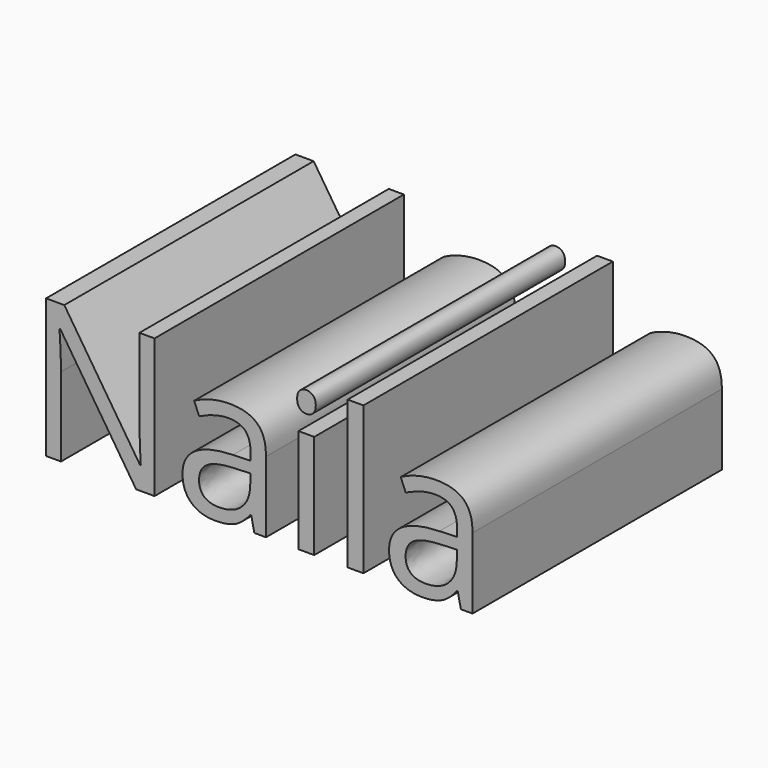
from build123d import *

# Parameters (mm, degrees)
F0_TEXT_SIZE = 15.8483641119
F1_DEPTH     = 25.4


# Not quite as in the source:
# - Text() gives the source's letters only with a copy of the font that has no kerning and outlines rounded to 1/6400 em; it was checked with that copy


with BuildPart() as f1:
    # F0 (on Front) → F1 (new body)
    with BuildSketch(Plane.XZ):
        with Locations((-37.3377553248, 0)):
            Text('Naila', F0_TEXT_SIZE, font='Open Sans', text_align=(TextAlign.LEFT, TextAlign.BOTTOM))
    extrude(amount=F1_DEPTH)


solid = f1.part
